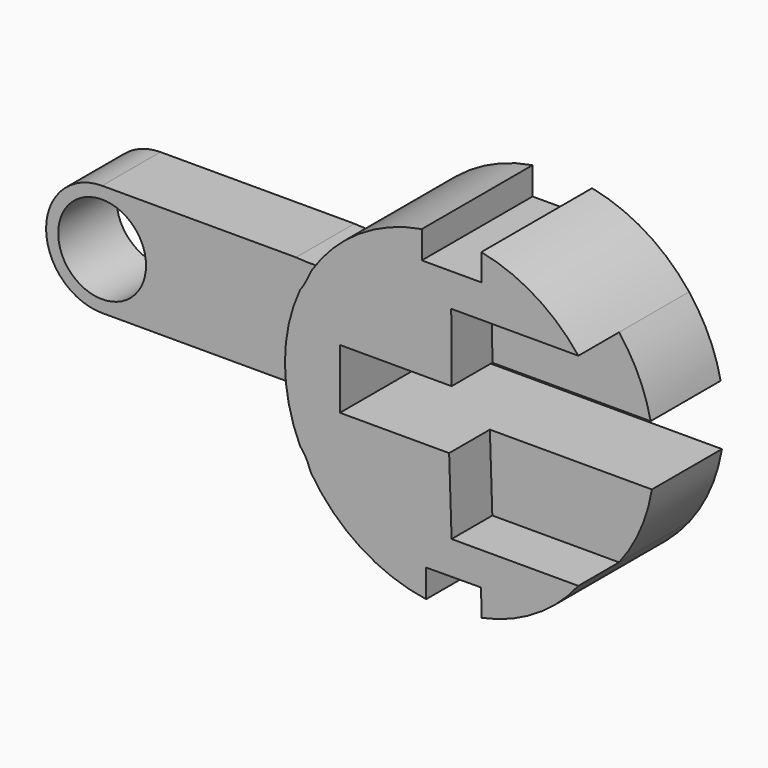
from build123d import *

# Parameters (mm, degrees)
F0_R     = 6.1702881354
F1_DEPTH = 10.24551
F2_DEPTH = 19.44125
F3_DEPTH = 12.29025


# Not quite as in the source:
# - the program builds the solid bodies; features that only make, move or delete a surface that nothing else refers to are left out


with BuildPart() as f1:
    # F0 (on Front) → F1 (new body)
    with BuildSketch(Plane.XZ):
        with BuildLine():
            ThreePointArc((7.9096967883, -9.6482263274), (5.7944386046, 0), (7.9096967883, 9.6482263274))
            add(Edge.make_bspline(
                [(7.9096967883, 9.6482263274), (7.1691805882, 8.7133229845), (4.8849042306, 7.0496072248), (1.7047020698, 7.2518519174), (0, 7.3653594591)],
                knots=[0.305255717, 0.305255717, 0.305255717, 0.305255717, 0.6293542053, 1, 1, 1, 1], degree=3))
            Line((0, 7.3653594591), (-27.2417403758, 7.3653594591))
            ThreePointArc((-27.2417403758, 7.3653594591), (-35.1115765516, -0.5044767167), (-27.2417403758, -8.3743128926))
            Line((-27.2417403758, -8.3743128926), (0, -8.3743128926))
            add(Edge.make_bspline(
                [(7.9096967883, -9.6482263274), (7.1553998901, -8.8616436412), (4.7881379326, -7.7629787373), (1.6803783566, -8.1685536627), (0, -8.3743128926)],
                knots=[0.3094407552, 0.3094407552, 0.3094407552, 0.3094407552, 0.6242726729, 1, 1, 1, 1], degree=3))
        make_face()
        with Locations((-27.2417403758, -0.5044767167)):
            Circle(F0_R, mode=Mode.SUBTRACT)
    extrude(amount=F1_DEPTH)

    # F0 (on Front) → F2 (join)
    with BuildSketch(Plane.XZ):
        with BuildLine():
            Line((29.1485549066, 14.2256355643), (47.0073711523, 14.2256355643))
            ThreePointArc((47.0073711523, 14.2256355643), (40.9442597431, 19.6396071394), (33.3793842605, 22.6136728933))
            Line((33.3793842605, 22.6136728933), (33.3793842605, 18.8674259181))
            Line((33.3793842605, 18.8674259181), (25.0220429152, 18.8674259181))
            Line((25.0220429152, 18.8674259181), (25.0220429152, 22.7406880158))
            ThreePointArc((25.0220429152, 22.7406880158), (16.1840833933, 19.2680953065), (9.494543791, 12.5287712643))
            add(Edge.make_bspline(
                [(9.494543791, 12.5287712643), (9.0162268309, 11.5501776901), (8.6071600956, 10.5287752978), (7.9096967883, 9.6482263274)],
                knots=[0, 0, 0, 0, 0.305255717, 0.305255717, 0.305255717, 0.305255717], degree=3))
            ThreePointArc((7.9096967883, 9.6482263274), (5.7944386046, 0), (7.9096967883, -9.6482263274))
            add(Edge.make_bspline(
                [(9.494543791, -12.5287712643), (9.0785331078, -11.4704442228), (8.6510771527, -10.4213396199), (7.9096967883, -9.6482263274)],
                knots=[0, 0, 0, 0, 0.3094407552, 0.3094407552, 0.3094407552, 0.3094407552], degree=3))
            ThreePointArc((9.494543791, -12.5287712643), (16.441223865, -19.434771268), (25.6276700044, -22.8345370586))
            Line((25.6276700044, -22.8345370586), (25.6276700044, -18.9136881421))
            Line((25.6276700044, -18.9136881421), (33.3589574797, -18.8714867898))
            Line((33.3589574797, -18.8714867898), (33.3793842605, -22.6136728933))
            ThreePointArc((33.3793842605, -22.6136728933), (40.9439316742, -19.6398090623), (47.0068958817, -14.2262419686))
            Line((47.0068958817, -14.2262419686), (29.2007135878, -14.2262419686))
            Line((29.2007135878, -14.2262419686), (28.8560651243, -3.7142947274))
            Line((28.8560651243, -3.7142947274), (13.5199762881, -3.7142947274))
            Line((13.5199762881, -3.7142947274), (13.5199762881, 4.6701654948))
            Line((13.5199762881, 4.6701654948), (29.2007135878, 4.6701654948))
            Line((29.2007135878, 4.6701654948), (29.1485549066, 14.2256355643))
        make_face()
    extrude(amount=F2_DEPTH)

    # F0 (on Front) → F3 (join)
    with BuildSketch(Plane.XZ):
        with BuildLine():
            ThreePointArc((47.0068958817, -14.2262419686), (49.9762101479, -9.2616462852), (51.6166150388, -3.7142947274))
            Line((51.6166150388, -3.7142947274), (28.8560651243, -3.7142947274))
            Line((28.8560651243, -3.7142947274), (29.2007135878, -14.2262419686))
            Line((29.2007135878, -14.2262419686), (47.0068958817, -14.2262419686))
        make_face()
        with BuildLine():
            Line((29.2007135878, 4.6701654948), (51.4398684351, 4.6701654948))
            ThreePointArc((51.4398684351, 4.6701654948), (49.7764866132, 9.704358941), (47.0073711523, 14.2256355643))
            Line((47.0073711523, 14.2256355643), (29.1485549066, 14.2256355643))
            Line((29.1485549066, 14.2256355643), (29.2007135878, 4.6701654948))
        make_face()
    extrude(amount=F3_DEPTH)


solid = f1.part
